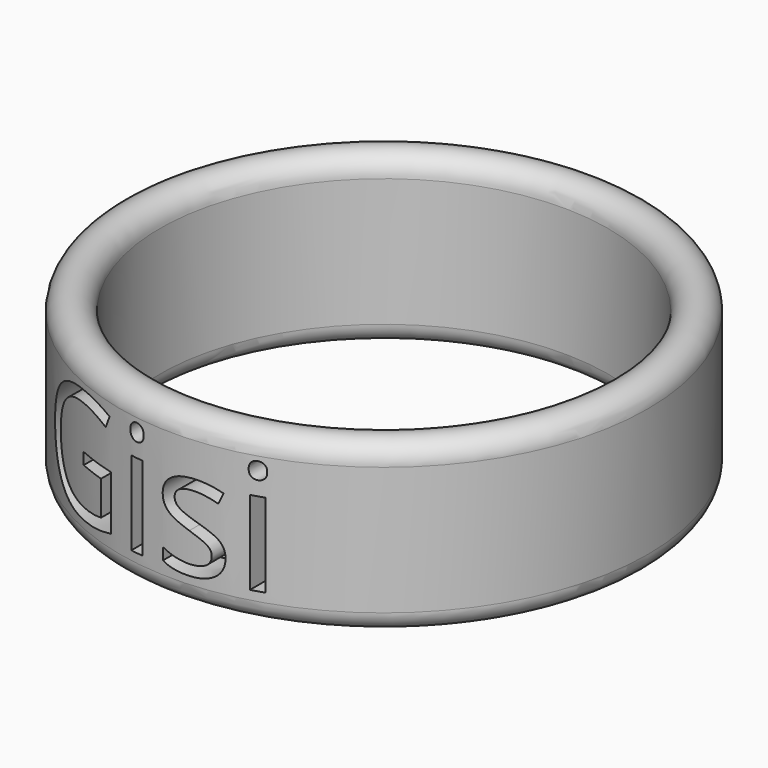
from build123d import *

# Parameters (mm, degrees)
F2_TEXT_SIZE = 24.3929874462
F3_DEPTH     = 107


# Not quite as in the source:
# - Text() gives the source's letters only with a copy of the font that has no kerning and outlines rounded to 1/6400 em; it was checked with that copy


with BuildPart() as f1:
    # F0 (on Front) → F1 (revolve)
    with BuildSketch(Plane.XZ):
        with BuildLine():
            ThreePointArc((41.2162803113, 10.2270678431), (38.1002724171, 13.3430757374), (34.9842645228, 10.2270678431))
            Line((34.9842645228, 10.2270678431), (34.9842645228, -9.7729321569))
            ThreePointArc((34.9842645228, -9.7729321569), (38.1002724171, -12.8889400512), (41.2162803113, -9.7729321569))
            Line((41.2162803113, -9.7729321569), (41.2162803113, 10.2270678431))
        make_face()
    revolve(axis=Axis((0, 0, -2.9071513563), (0, 0, 1)))

    # F2 (on Front) → F3 (cut)
    with BuildSketch(Plane.XZ):
        with Locations((-26.769336313, -8.3565656096)):
            Text('Gisi', F2_TEXT_SIZE, font='Open Sans', text_align=(TextAlign.LEFT, TextAlign.BOTTOM))
    extrude(amount=F3_DEPTH, mode=Mode.SUBTRACT)


solid = f1.part
